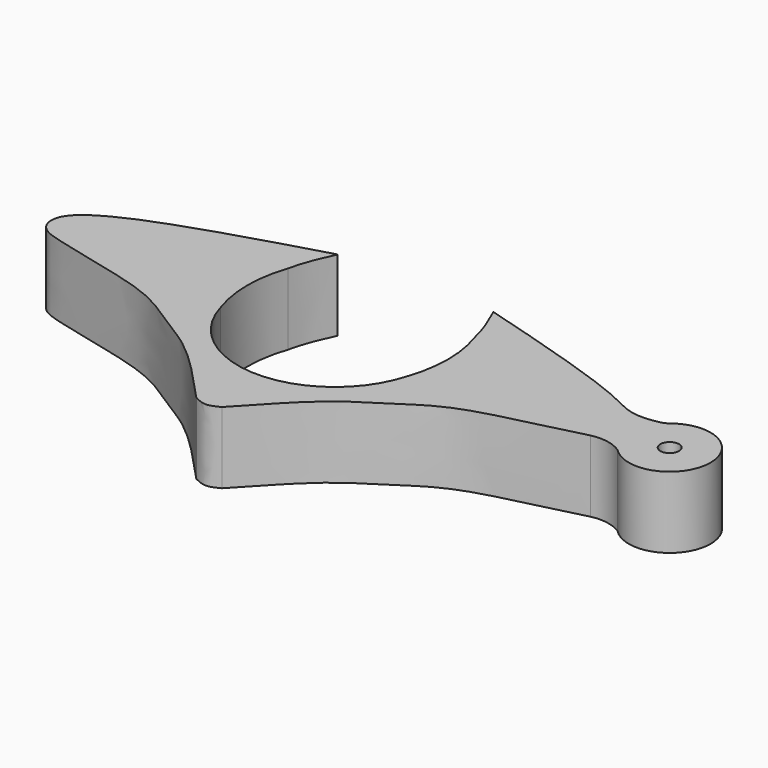
from build123d import *

# Parameters (mm, degrees)
F0_R     = 1.4985630317
F1_DEPTH = 11.43


with BuildPart() as f1:
    # F0 (on Top) → F1 (new body)
    with BuildSketch(Plane.XY):
        with BuildLine():
            add(Edge.make_bspline(
                [(-2.0359231176, -25.1206368319), (-1.3572468606, -25.4594553442), (0, -26.1375400989), (1.3572468606, -25.4594553442), (2.0359231176, -25.1206368319)],
                knots=[0, 0, 0, 0, 0.5, 1, 1, 1, 1], degree=3))
            add(Edge.make_bspline(
                [(2.0359231176, -25.1206368319), (3.3457383083, -23.7289975008), (5.9176088554, -20.9942341783), (8.3825547389, -18.3420624619), (12.9862326993, -14.1723402798), (17.2483349718, -11.8697604881), (23.5822979488, -7.1258779534), (33.3196303031, -4.7357772117), (39.6236724826, -3.217253521), (42.3201246069, -2.5082482566), (42.7449258083, -2.3794347429)],
                knots=[0.0267318689, 0.0267318689, 0.0267318689, 0.0267318689, 0.0793940725, 0.1368856043, 0.2045627996, 0.2663300013, 0.3434968825, 0.4325298389, 0.5123744144, 0.5283607708, 0.5283607708, 0.5283607708, 0.5283607708], degree=3))
            add(Edge.make_bspline(
                [(42.7449258083, -2.3794347429), (43.8815731542, -2.0347663711), (46.045577935, -1.0853188279), (46.5822686786, 2.7847802254), (43.1373679174, 5.284193473), (40.9767322457, 6.4169524924)],
                knots=[0.5283607708, 0.5283607708, 0.5283607708, 0.5283607708, 0.5711357195, 0.6250302421, 0.6734394222, 0.6734394222, 0.6734394222, 0.6734394222], degree=3))
            ThreePointArc((40.9767322457, 6.4169524924), (40.8675160296, 6.4727238237), (40.7590710313, 6.5299803131))
            add(Edge.make_bspline(
                [(40.7590710313, 6.5299803131), (37.6023937497, 8.1537861369), (27.6170269646, 11.7427429089), (17.0369422947, 14.7816914556), (12.4444465447, 16.107118844)],
                knots=[0.6750518947, 0.6750518947, 0.6750518947, 0.6750518947, 0.7446505875, 0.8393118979, 0.8393118979, 0.8393118979, 0.8393118979], degree=3))
            add(Edge.make_bspline(
                [(12.4444465447, 16.107118844), (13.4288124201, 13.9138079535), (14.405733434, 11.706479395), (14.9060189724, 9.307032451)],
                knots=[0, 0, 0, 0, 0.4869217945, 0.4869217945, 0.4869217945, 0.4869217945], degree=3))
            ThreePointArc((14.9060189724, 9.307032451), (16.033692156, 2.5682199114), (14.9060189724, -4.1705926282))
            ThreePointArc((14.9060189724, -4.1705926282), (0, -15.4784768138), (-14.9060189724, -4.1705926282))
            ThreePointArc((-14.9060189724, -4.1705926282), (-16.033692156, 2.5682199114), (-14.9060189724, 9.307032451))
            add(Edge.make_bspline(
                [(-12.4444465447, 16.107118844), (-13.4288124201, 13.9138079535), (-14.405733434, 11.706479395), (-14.9060189724, 9.307032451)],
                knots=[0, 0, 0, 0, 0.4869217945, 0.4869217945, 0.4869217945, 0.4869217945], degree=3))
            add(Edge.make_bspline(
                [(-2.0359231176, -25.1206368319), (-3.3457383083, -23.7289975008), (-5.9176088554, -20.9942341783), (-8.3825547389, -18.3420624619), (-12.9862326993, -14.1723402798), (-17.2483349718, -11.8697604881), (-23.5822979488, -7.1258779534), (-33.3196303031, -4.7357772117), (-41.0823407103, -2.8658881275), (-45.9864394649, -1.5117687719), (-46.8457007748, 4.6843999202), (-30.8389514135, 10.8173001618), (-17.0369422947, 14.7816914556), (-12.4444465447, 16.107118844)],
                knots=[0.0267318689, 0.0267318689, 0.0267318689, 0.0267318689, 0.0793940725, 0.1368856043, 0.2045627996, 0.2663300013, 0.3434968825, 0.4325298389, 0.5123744144, 0.5711357195, 0.6250302421, 0.7446505875, 0.8393118979, 0.8393118979, 0.8393118979, 0.8393118979], degree=3))
        make_face()
        with BuildLine():
            add(Edge.make_bspline(
                [(42.7449258083, -2.3794347429), (43.8815731542, -2.0347663711), (46.045577935, -1.0853188279), (46.5822686786, 2.7847802254), (43.1373679174, 5.284193473), (40.9767322457, 6.4169524924)],
                knots=[0.5283607708, 0.5283607708, 0.5283607708, 0.5283607708, 0.5711357195, 0.6250302421, 0.6734394222, 0.6734394222, 0.6734394222, 0.6734394222], degree=3))
            ThreePointArc((42.7449258083, -2.3794347429), (45.378860283, -2.3288884868), (47.8265587579, -3.3030229318))
            ThreePointArc((47.8265587579, -3.3030229318), (58.9944758829, 0.412176161), (49.1102670664, 6.8018156877))
            ThreePointArc((49.1102670664, 6.8018156877), (48.3608651105, 6.266695872), (47.5288443445, 5.8721100719))
            ThreePointArc((47.5288443445, 5.8721100719), (45.6991604767, 5.5642789991), (43.843957286, 5.5373690255))
            ThreePointArc((43.843957286, 5.5373690255), (42.3733924319, 5.8567052695), (40.9767322457, 6.4169524924))
        make_face()
        with Locations((52.5188855827, 1.2348284946)):
            Circle(F0_R, mode=Mode.SUBTRACT)
    extrude(amount=F1_DEPTH)


solid = f1.part
